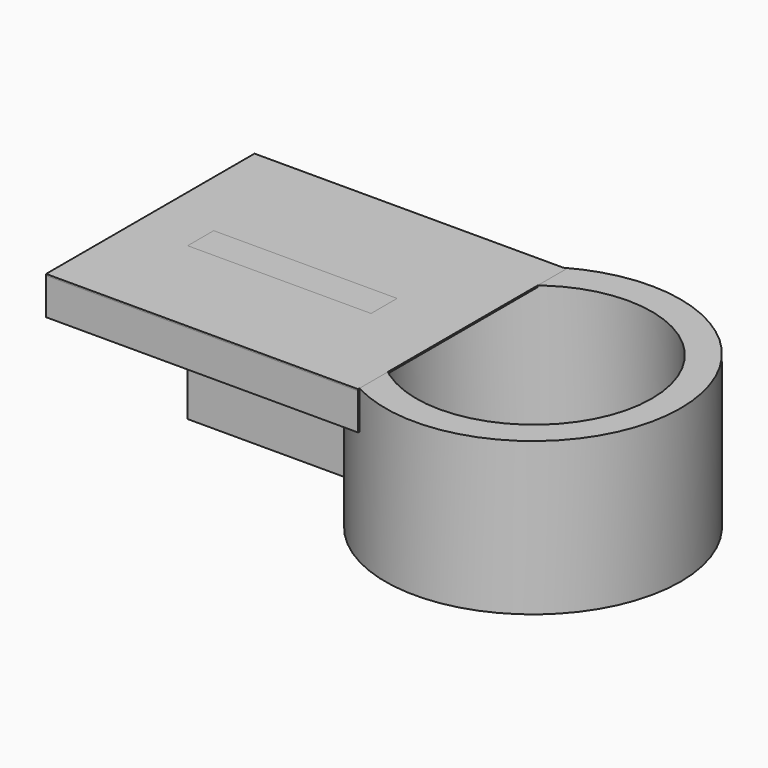
from build123d import *

# Parameters (mm, degrees)
F0_W     = 51.9137978554
F0_H     = 43.3565778658
F1_DEPTH = 6.35
F2_R     = 24.5600108098
F3_DEPTH = 25.4
F4_R     = 19.6018385594
F5_DEPTH = 43.18
F6_DEPTH = 0.254
F7_W     = 30.5207502097
F7_H     = 5.4195709527
F8_DEPTH = 25.4


# Not quite as in the source:
# - a feature of the source that left no trace in its solid (it failed there, or was rolled back) is left out


with BuildPart() as f1:
    # F0 (on Top) → F1 (new body)
    with BuildSketch(Plane.XY):
        with Locations((-25.9568989277, 29.522406403)):
            Rectangle(F0_W, F0_H)
    extrude(amount=-F1_DEPTH)

    # F2 (on Top) → F3 (join)
    with BuildSketch(Plane.XY):
        with Locations((11.5432187769, 29.8076476902)):
            Circle(F2_R)
    extrude(amount=-F3_DEPTH)

    # F4 (on Top) → F5 (cut)
    with BuildSketch(Plane.XY):
        with Locations((11.8770356263, 29.6167964683)):
            Circle(F4_R)
    extrude(amount=-F5_DEPTH, mode=Mode.SUBTRACT)


with BuildPart() as f6:
    # F0 (on Top) → F6 (new body)
    with BuildSketch(Plane.XY):
        with Locations((-25.9568989277, 29.522406403)):
            Rectangle(F0_W, F0_H)
    extrude(amount=-F6_DEPTH)


with BuildPart() as f8:
    # F7 (on Top) → F8 (new body)
    with BuildSketch(Plane.XY):
        with Locations((-27.240482159, 28.2388236374)):
            Rectangle(F7_W, F7_H)
    extrude(amount=-F8_DEPTH)


solid = Compound([f1.part, f6.part, f8.part])
